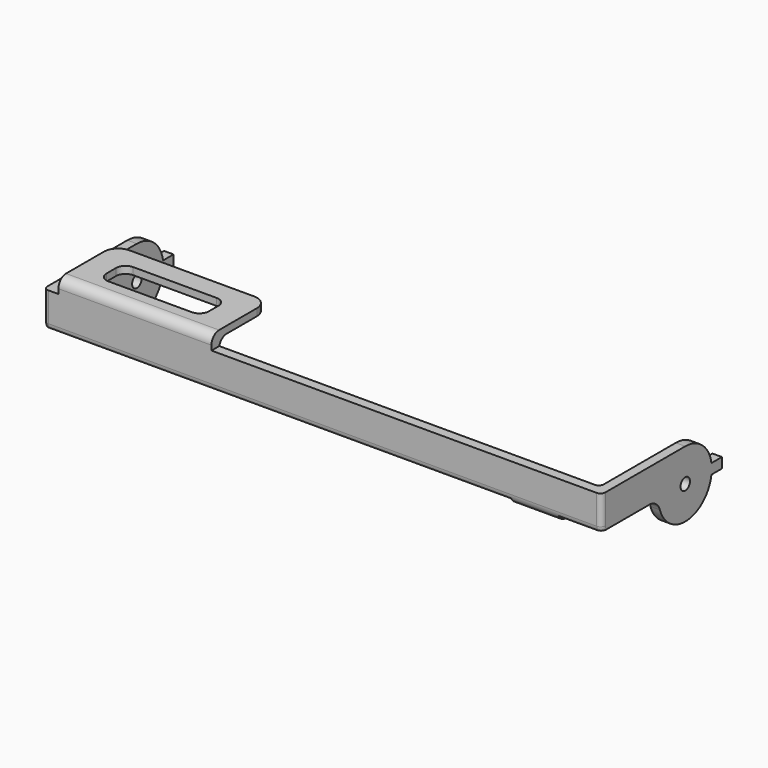
from build123d import *

# Parameters (mm, degrees)
F1_DEPTH  = 7
F2_R      = 7
F3_DEPTH  = 2
F4_R      = 7
F5_DEPTH  = 2
F6_W      = 32.3093086481
F6_H      = 2
F7_DEPTH  = 3
F8_W      = 32.3093086481
F8_H      = 1.5
F9_DEPTH  = 13
F11_W     = 10
F11_H     = 1.2
F12_DEPTH = 10
F13_DEPTH = 25
F14_R     = 3
F15_R     = 2
F16_R     = 1
F17_DEPTH = 117.7887811979
F18_R     = 3
F19_W     = 5.0336755812
F19_H     = 2.1570066456
F20_DEPTH = 2
F22_DEPTH = 2
F23_D     = 2.5


with BuildPart() as f1:
    # F0 (on Top) → F1 (new body)
    with BuildSketch(Plane.XY):
        Polygon((-114.8008331656, 27.8736967593), (-116.8008331656, 27.8736967593), (-116.8008331656, -1.2305311393), (0.9869479323, -1.2305311393), (0.9869479323, 27.8736967593), (-1.0130520677, 27.8736967593), (-1.0130520677, 0.7694688607), (-114.8008331656, 0.7694688607), align=None)
    extrude(amount=F1_DEPTH)

    # F2 (on face) → F3 (join)
    with BuildSketch(Plane(origin=(-116.8008331656, 0, 0), x_dir=(0, -1, 0), z_dir=(-1, 0, 0))):
        with Locations((-20.8736967593, 0)):
            Circle(F2_R)
    extrude(amount=-F3_DEPTH)

    # F4 (on face) → F5 (join)
    with BuildSketch(Plane(origin=(-1.0130520677, 0, 0), x_dir=(0, -1, 0), z_dir=(-1, 0, 0))):
        with Locations((-20.8736967593, 0)):
            Circle(F4_R)
    extrude(amount=-F5_DEPTH)

    # F6 (on face) → F7 (join)
    with BuildSketch(Plane.XY.offset(7)):
        with Locations((-97.5135117769, -0.2305311393)):
            Rectangle(F6_W, F6_H)
    extrude(amount=F7_DEPTH)

    # F8 (on face) → F9 (join)
    with BuildSketch(Plane(origin=(0, 0.7694688607, 0), x_dir=(-1, 0, 0), z_dir=(0, 1, 0))):
        with Locations((97.5135117769, 9.25)):
            Rectangle(F8_W, F8_H)
    extrude(amount=F9_DEPTH)

    # F11 (on face) → F12 (join)
    with BuildSketch(Plane.XZ.offset(1.2305311393)):
        with Locations((-13.2145643048, -0.6)):
            Rectangle(F11_W, F11_H)
    extrude(amount=-F12_DEPTH)

    # F10 (on face) → F13 (cut)
    with BuildSketch(Plane.XY.offset(10)):
        with BuildLine():
            ThreePointArc((-86.8486179709, 7.4843045808), (-87.4344044086, 8.8985181432), (-88.8486179709, 9.4843045808))
            Line((-88.8486179709, 9.4843045808), (-106.4697470069, 9.4843045808))
            ThreePointArc((-106.4697470069, 9.4843045808), (-107.8839605693, 8.8985181432), (-108.4697470069, 7.4843045808))
            Line((-108.4697470069, 7.4843045808), (-108.4697470069, 4.9521672986))
            ThreePointArc((-108.4697470069, 4.9521672986), (-108.4179393254, 4.4998989157), (-108.2652003167, 4.0710615092))
            ThreePointArc((-108.2652003167, 4.0710615092), (-107.9372939182, 3.5933788445), (-107.4862224218, 3.2297336335))
            ThreePointArc((-107.4862224218, 3.2297336335), (-106.996592653, 3.0228063513), (-106.4697470069, 2.9521672986))
            Line((-106.4697470069, 2.9521672986), (-88.8486179709, 2.9521672986))
            ThreePointArc((-88.8486179709, 2.9521672986), (-87.4344044086, 3.5379537363), (-86.8486179709, 4.9521672986))
            Line((-86.8486179709, 4.9521672986), (-86.8486179709, 7.4843045808))
        make_face()
    extrude(amount=-F13_DEPTH, mode=Mode.SUBTRACT)

    # F14
    f14_edges = [f1.edges().sort_by_distance(p)[0] for p in [
        (-113.668166, 13.769469, 9.25),
        (-81.358857, 13.769469, 9.25),
    ]]
    fillet(f14_edges, radius=F14_R)

    # F15
    f15_edges = [f1.edges().sort_by_distance(p)[0] for p in [
        (-97.513512, -1.230531, 10),
        (-97.513512, 0.769469, 8.5),
        (-13.214564, -1.230531, -1.2),
    ]]
    fillet(f15_edges, radius=F15_R)

    # F16
    f16_edges = [f1.edges().sort_by_distance(p)[0] for p in [
        (-13.214564, 0.769469, 0),
        (-1.013052, 0.769469, 3.25),
        (0.986948, -1.230531, 3.9),
        (-116.800833, -1.230531, 3.9),
        (-114.800833, 0.769469, 3.25),
        (-18.214564, 8.769469, -0.6),
        (-8.214564, 8.769469, -0.6),
        (-1.013052, 0.785409, 6.752009),
        (-114.800833, 0.785409, 6.752009),
        (-116.800833, -1.188344, 0.391381),
        (0.986948, -1.188344, 0.391381),
    ]]
    fillet(f16_edges, radius=F16_R)

    # F2 (on face) → F17 (cut, through all)
    with BuildSketch(Plane(origin=(-116.8008331656, 0, 0), x_dir=(0, -1, 0), z_dir=(-1, 0, 0))):
        with BuildLine():
            Line((-27.8736967593, 7), (-27.8736967593, 0))
            ThreePointArc((-27.8736967593, 0), (-25.8234442276, 4.9497474683), (-20.8736967593, 7))
            Line((-20.8736967593, 7), (-27.8736967593, 7))
        make_face()
    extrude(amount=-F17_DEPTH, mode=Mode.SUBTRACT)

    # F18
    f18_edges = [f1.edges().sort_by_distance(p)[0] for p in [
        (-115.800833, 13.873697, 0),
        (-0.013052, 13.873697, 0),
    ]]
    fillet(f18_edges, radius=F18_R)

    # F19 (on face) → F20 (join)
    with BuildSketch(Plane(origin=(-116.8008331656, 0, 0), x_dir=(0, -1, 0), z_dir=(-1, 0, 0))):
        with Locations((-28.0387327075, 0)):
            Rectangle(F19_W, F19_H)
    extrude(amount=-F20_DEPTH)

    # F21 (on face) → F22 (join)
    with BuildSketch(Plane(origin=(-1.0130520677, 0, 0), x_dir=(0, -1, 0), z_dir=(-1, 0, 0))):
        with BuildLine():
            Line((-27.7901142267, 1.0785033228), (-30.5555704981, 1.0785033228))
            Line((-30.5555704981, 1.0785033228), (-30.5555704981, -1.0785033228))
            Line((-30.5555704981, -1.0785033228), (-27.7901142267, -1.0785033228))
            ThreePointArc((-27.7901142267, -1.0785033228), (-27.8736967593, 0), (-27.7901142267, 1.0785033228))
        make_face()
    extrude(amount=-F22_DEPTH)

    # F23 (through all)
    with Locations(Plane(origin=(-116.8008331656, 0, 0), x_dir=(0, -1, 0), z_dir=(-1, 0, 0))):
        with Locations((-20.8736967593, 0)):
            Hole(F23_D / 2)


solid = f1.part
